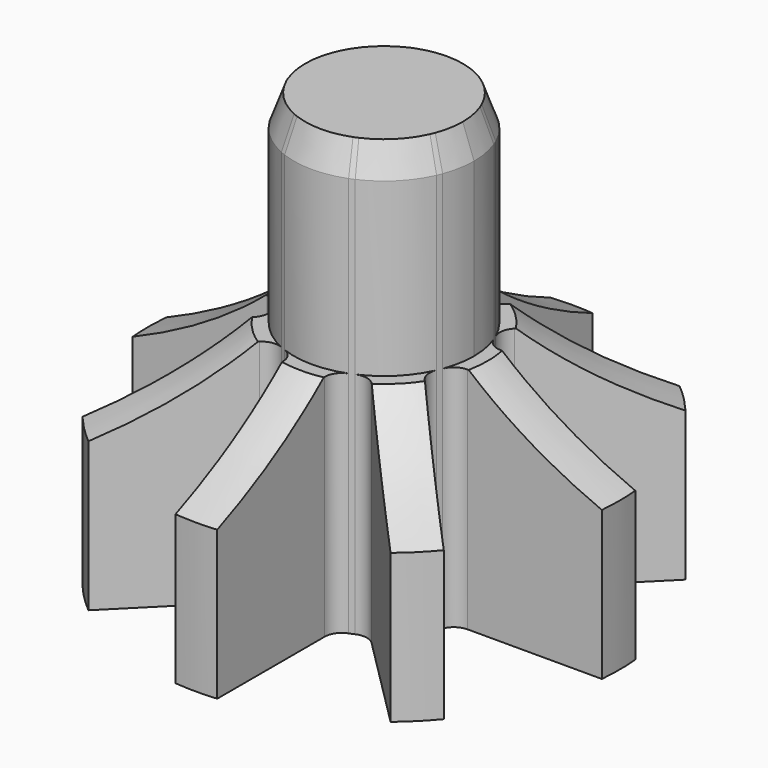
from build123d import *

# Parameters (mm, degrees)
F0_R      = 58.42
F1_DEPTH  = 10.16
F2_R      = 58.42
F2_R_2    = 36.83
F3_DEPTH  = 0.4
F7_DEPTH  = 9
F8_R      = 74.9748378887
F8_R_2    = 10.4599607608
F9_DEPTH  = 19.161
F10_SIZE2 = 1.3737387097
F10_SIZE  = 0.5


# Not quite as in the source:
# - a feature names something its author has since deleted; it is built from what else it names


with BuildPart() as f1:
    # F0 (on Top) → F1 (new body)
    with BuildSketch(Plane.XY):
        Circle(F0_R)
        with BuildLine():
            ThreePointArc((-0.9277419355, -57.1424692755), (-21.8703581597, -52.799715283), (-39.7498149047, -41.0618401322))
            Line((-39.7498149047, -41.0618401322), (-27.1737640713, -28.4857892989))
            Line((-27.1737640713, -28.4857892989), (-2.492115099, -3.8041403265))
            ThreePointArc((-2.492115099, -3.8041403265), (-2.0907477912, -3.5934545057), (-1.6407389599, -3.6480098226))
            ThreePointArc((-1.6407389599, -3.6480098226), (-1.5307337295, -3.69551813), (-1.4193548387, -3.739710128))
            ThreePointArc((-1.4193548387, -3.739710128), (-1.062574108, -4.0193379897), (-0.9277419355, -4.4521249074))
            Line((-0.9277419355, -4.4521249074), (-0.9277419355, -38.0870768925))
            Line((-0.9277419355, -38.0870768925), (-0.9277419355, -57.1424692755))
        make_face(mode=Mode.SUBTRACT)
        with BuildLine():
            ThreePointArc((-41.0618401322, -39.7498149047), (-52.799715283, -21.8703581597), (-57.1424692755, -0.9277419355))
            Line((-57.1424692755, -0.9277419355), (-39.3572476259, -0.9277419355))
            Line((-39.3572476259, -0.9277419355), (-4.4521249074, -0.9277419355))
            ThreePointArc((-4.4521249074, -0.9277419355), (-4.0193379897, -1.062574108), (-3.739710128, -1.4193548387))
            ThreePointArc((-3.739710128, -1.4193548387), (-3.69551813, -1.5307337295), (-3.6480098226, -1.6407389599))
            ThreePointArc((-3.6480098226, -1.6407389599), (-3.5934545057, -2.0907477912), (-3.8041403265, -2.492115099))
            Line((-3.8041403265, -2.492115099), (-27.5876429601, -26.2756177325))
            Line((-27.5876429601, -26.2756177325), (-41.0618401322, -39.7498149047))
        make_face(mode=Mode.SUBTRACT)
        with BuildLine():
            ThreePointArc((39.7498149047, -41.0618401322), (21.8703581597, -52.799715283), (0.9277419355, -57.1424692755))
            Line((0.9277419355, -57.1424692755), (0.9277419355, -39.3572476259))
            Line((0.9277419355, -39.3572476259), (0.9277419355, -4.4521249074))
            ThreePointArc((0.9277419355, -4.4521249074), (1.062574108, -4.0193379897), (1.4193548387, -3.739710128))
            ThreePointArc((1.4193548387, -3.739710128), (1.5307337295, -3.69551813), (1.6407389599, -3.6480098226))
            ThreePointArc((1.6407389599, -3.6480098226), (2.0907477912, -3.5934545057), (2.492115099, -3.8041403265))
            Line((2.492115099, -3.8041403265), (27.1737640713, -28.4857892989))
            Line((27.1737640713, -28.4857892989), (39.7498149047, -41.0618401322))
        make_face(mode=Mode.SUBTRACT)
        with BuildLine():
            ThreePointArc((57.1424692755, -0.9277419355), (52.799715283, -21.8703581597), (41.0618401322, -39.7498149047))
            Line((41.0618401322, -39.7498149047), (27.5876429601, -26.2756177325))
            Line((27.5876429601, -26.2756177325), (3.8041403265, -2.492115099))
            ThreePointArc((3.8041403265, -2.492115099), (3.5934545057, -2.0907477912), (3.6480098226, -1.6407389599))
            ThreePointArc((3.6480098226, -1.6407389599), (3.69551813, -1.5307337295), (3.739710128, -1.4193548387))
            ThreePointArc((3.739710128, -1.4193548387), (4.0193379897, -1.062574108), (4.4521249074, -0.9277419355))
            Line((4.4521249074, -0.9277419355), (38.0870768925, -0.9277419355))
            Line((38.0870768925, -0.9277419355), (57.1424692755, -0.9277419355))
        make_face(mode=Mode.SUBTRACT)
        with BuildLine():
            ThreePointArc((-3.8041403265, 2.492115099), (-3.5934545057, 2.0907477912), (-3.6480098226, 1.6407389599))
            ThreePointArc((-3.6480098226, 1.6407389599), (-3.69551813, 1.5307337295), (-3.739710128, 1.4193548387))
            ThreePointArc((-3.739710128, 1.4193548387), (-4.0193379897, 1.062574108), (-4.4521249074, 0.9277419355))
            Line((-4.4521249074, 0.9277419355), (-38.0870768925, 0.9277419355))
            Line((-38.0870768925, 0.9277419355), (-57.1424692755, 0.9277419355))
            ThreePointArc((-57.1424692755, 0.9277419355), (-52.799715283, 21.8703581597), (-41.0618401322, 39.7498149047))
            Line((-41.0618401322, 39.7498149047), (-27.5876429601, 26.2756177325))
            Line((-27.5876429601, 26.2756177325), (-3.8041403265, 2.492115099))
        make_face(mode=Mode.SUBTRACT)
        with BuildLine():
            ThreePointArc((-39.7498149047, 41.0618401322), (-21.8703581597, 52.799715283), (-0.9277419355, 57.1424692755))
            Line((-0.9277419355, 57.1424692755), (-0.9277419355, 39.3572476259))
            Line((-0.9277419355, 39.3572476259), (-0.9277419355, 4.4521249074))
            ThreePointArc((-0.9277419355, 4.4521249074), (-1.062574108, 4.0193379897), (-1.4193548387, 3.739710128))
            ThreePointArc((-1.4193548387, 3.739710128), (-1.5307337295, 3.69551813), (-1.6407389599, 3.6480098226))
            ThreePointArc((-1.6407389599, 3.6480098226), (-2.0907477912, 3.5934545057), (-2.492115099, 3.8041403265))
            Line((-2.492115099, 3.8041403265), (-26.2756177325, 27.5876429601))
            Line((-26.2756177325, 27.5876429601), (-39.7498149047, 41.0618401322))
        make_face(mode=Mode.SUBTRACT)
        with BuildLine():
            ThreePointArc((41.0618401322, 39.7498149047), (52.799715283, 21.8703581597), (57.1424692755, 0.9277419355))
            Line((57.1424692755, 0.9277419355), (39.3572476259, 0.9277419355))
            Line((39.3572476259, 0.9277419355), (4.4521249074, 0.9277419355))
            ThreePointArc((4.4521249074, 0.9277419355), (4.0193379897, 1.062574108), (3.739710128, 1.4193548387))
            ThreePointArc((3.739710128, 1.4193548387), (3.69551813, 1.5307337295), (3.6480098226, 1.6407389599))
            ThreePointArc((3.6480098226, 1.6407389599), (3.5934545057, 2.0907477912), (3.8041403265, 2.492115099))
            Line((3.8041403265, 2.492115099), (28.4857892989, 27.1737640713))
            Line((28.4857892989, 27.1737640713), (41.0618401322, 39.7498149047))
        make_face(mode=Mode.SUBTRACT)
        with BuildLine():
            Line((0.9277419355, 38.0870768925), (0.9277419355, 57.1424692755))
            ThreePointArc((0.9277419355, 57.1424692755), (21.8703581597, 52.799715283), (39.7498149047, 41.0618401322))
            Line((39.7498149047, 41.0618401322), (26.2756177325, 27.5876429601))
            Line((26.2756177325, 27.5876429601), (2.492115099, 3.8041403265))
            ThreePointArc((2.492115099, 3.8041403265), (2.0907477912, 3.5934545057), (1.6407389599, 3.6480098226))
            ThreePointArc((1.6407389599, 3.6480098226), (1.5307337295, 3.69551813), (1.4193548387, 3.739710128))
            ThreePointArc((1.4193548387, 3.739710128), (1.062574108, 4.0193379897), (0.9277419355, 4.4521249074))
            Line((0.9277419355, 4.4521249074), (0.9277419355, 38.0870768925))
        make_face(mode=Mode.SUBTRACT)
    extrude(amount=F1_DEPTH)

    # F2 (on Top) → F3 (join)
    with BuildSketch(Plane.XY):
        Circle(F2_R)
        Circle(F2_R_2, mode=Mode.SUBTRACT)
    extrude(amount=F3_DEPTH)

    # F4 (on Right) → F5 (revolve, cut)
    with BuildSketch(Plane.YZ):
        with BuildLine():
            Line((59.8527193069, 24.0727756172), (0, 24.0727756172))
            Line((0, 24.0727756172), (0, 16.6299855337))
            add(Edge.make_bspline(
                [(0, 16.6299855337), (1.5682306201, 12.4801510163), (11.0409046545, 1.6871235144), (51.8005160159, 3.1310333802), (58.4798612628, 1.06584979), (59.8527193069, 0)],
                knots=[0, 0, 0, 0, 0.3076669633, 0.789053117, 1, 1, 1, 1], degree=3))
            Line((59.8527193069, 0), (59.8527193069, 24.0727756172))
        make_face()
    revolve(axis=Axis((0, 0, 0), (0, 0, -1)), mode=Mode.SUBTRACT)

    # F6 (on face) → F7 (join)
    with BuildSketch(Plane.XY.offset(10.16)):
        with BuildLine():
            ThreePointArc((3.739710128, -1.4193548387), (3.9343894388, -0.7215121232), (4, 0))
            ThreePointArc((4, 0), (3.9343894388, 0.7215121232), (3.739710128, 1.4193548387))
            ThreePointArc((3.739710128, 1.4193548387), (3.69551813, 1.5307337295), (3.6480098226, 1.6407389599))
            ThreePointArc((3.6480098226, 1.6407389599), (2.8284271247, 2.8284271247), (1.6407389599, 3.6480098226))
            ThreePointArc((1.6407389599, 3.6480098226), (1.5307337295, 3.69551813), (1.4193548387, 3.739710128))
            ThreePointArc((1.4193548387, 3.739710128), (0, 4), (-1.4193548387, 3.739710128))
            ThreePointArc((-1.4193548387, 3.739710128), (-1.5307337295, 3.69551813), (-1.6407389599, 3.6480098226))
            ThreePointArc((-1.6407389599, 3.6480098226), (-2.8284271247, 2.8284271247), (-3.6480098226, 1.6407389599))
            ThreePointArc((-3.6480098226, 1.6407389599), (-3.69551813, 1.5307337295), (-3.739710128, 1.4193548387))
            ThreePointArc((-3.739710128, 1.4193548387), (-4, 0), (-3.739710128, -1.4193548387))
            ThreePointArc((-3.739710128, -1.4193548387), (-3.69551813, -1.5307337295), (-3.6480098226, -1.6407389599))
            ThreePointArc((-3.6480098226, -1.6407389599), (-2.8284271247, -2.8284271247), (-1.6407389599, -3.6480098226))
            ThreePointArc((-1.6407389599, -3.6480098226), (-1.5307337295, -3.69551813), (-1.4193548387, -3.739710128))
            ThreePointArc((-1.4193548387, -3.739710128), (0, -4), (1.4193548387, -3.739710128))
            ThreePointArc((1.4193548387, -3.739710128), (1.5307337295, -3.69551813), (1.6407389599, -3.6480098226))
            ThreePointArc((1.6407389599, -3.6480098226), (2.8284271247, -2.8284271247), (3.6480098226, -1.6407389599))
            ThreePointArc((3.6480098226, -1.6407389599), (3.69551813, -1.5307337295), (3.739710128, -1.4193548387))
        make_face()
    extrude(amount=F7_DEPTH)

    # F8 (on Top) → F9 (cut, through all)
    with BuildSketch(Plane.XY):
        Circle(F8_R)
        Circle(F8_R_2, mode=Mode.SUBTRACT)
    extrude(amount=F9_DEPTH, mode=Mode.SUBTRACT)

    # F10
    f10_edges = [f1.edges().sort_by_distance(p)[0] for p in [
        (-3.73971, 1.419355, 19.16),
    ]]
    f10_side = f1.faces().sort_by_distance((0, 0, 19.16))[0]
    chamfer(f10_edges, length=F10_SIZE, length2=F10_SIZE2, reference=f10_side)


solid = f1.part
